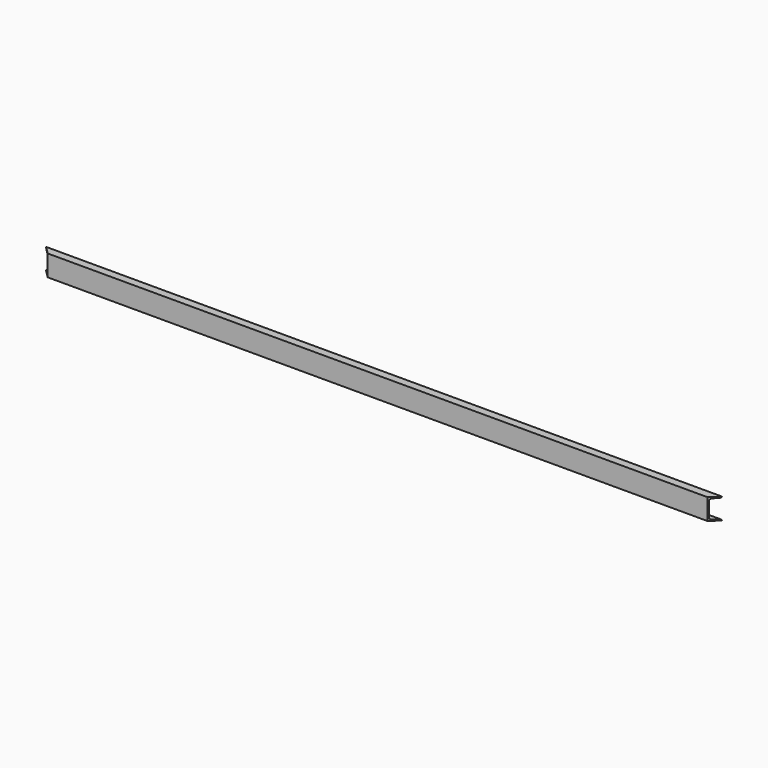
from build123d import *

# Parameters (mm, degrees)
F1_DEPTH = 6500
F3_DEPTH = 203.001


# Not quite as in the source:
# - a pattern or mirror of a feature is missing from the dataset's text; its kind, count and spacing are read off the source's solid


with BuildPart() as f1:
    # F0 (on Right) → F1 (new body)
    with BuildSketch(Plane.YZ):
        with BuildLine():
            Line((0, 203), (0, 0.7243087391))
            Line((0, 0.7243087391), (76, 0.7243087391))
            Line((76, 0.7243087391), (76, 2.0526619257))
            ThreePointArc((76, 2.0526619257), (73.6656821536, 7.9036758191), (67.9448556281, 10.5410129711))
            Line((67.9448556281, 10.5410129711), (23.2102887439, 12.8854522787))
            ThreePointArc((23.2102887439, 12.8854522787), (11.7686356928, 18.1601265828), (7.1, 29.8621543695))
            Line((7.1, 29.8621543695), (7.1, 173.8621543695))
            ThreePointArc((7.1, 173.8621543695), (11.7686356928, 185.5641821563), (23.2102887439, 190.8388564604))
            Line((23.2102887439, 190.8388564604), (67.9448556281, 193.183295768))
            ThreePointArc((67.9448556281, 193.183295768), (73.6656821536, 195.82063292), (76, 201.6716468134))
            Line((76, 201.6716468134), (76, 203))
            Line((76, 203), (0, 203))
        make_face()
    extrude(amount=F1_DEPTH)

    # F2 (on Top) → F3 (cut, through all)
    with BuildSketch(Plane.XY):
        Polygon((0, 76), (0, 0), (76, 0), align=None)
    f3 = extrude(amount=F3_DEPTH, mode=Mode.SUBTRACT)

    # F3_copies: F3 across plane
    add(f3.mirror(Plane(origin=(3250, 0, 0), x_dir=(0, 0, 1), z_dir=(1, 0, 0))), mode=Mode.SUBTRACT)


solid = f1.part
